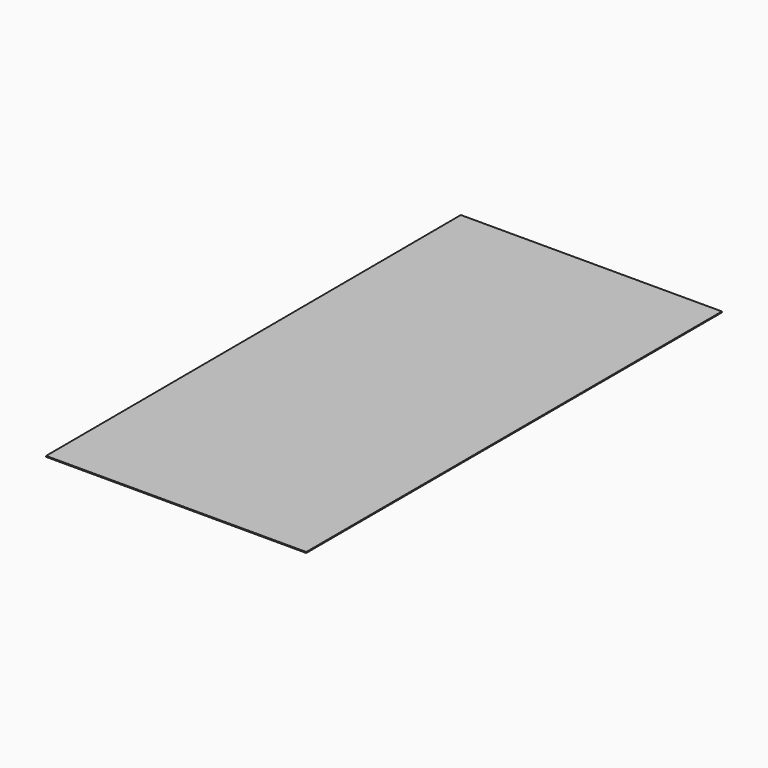
from build123d import *

# Parameters (mm, degrees)
F1_DEPTH = 3.175


# Not quite as in the source:
# - a length typed as a fraction of an inch, garbled in the dataset ("3 / 203.2 mm" for 3/8 in), is restored


with BuildPart() as f1:
    # F0 (on Top) → F1 (new body)
    with BuildSketch(Plane.XY):
        Polygon((-41.8675243855, 60.8982294798), (-36.3591299281, -1767.8934747858), (878.0408700719, -1767.8934747858), (875.7074756145, 60.8982294798), align=None)
    extrude(amount=F1_DEPTH)


solid = f1.part
